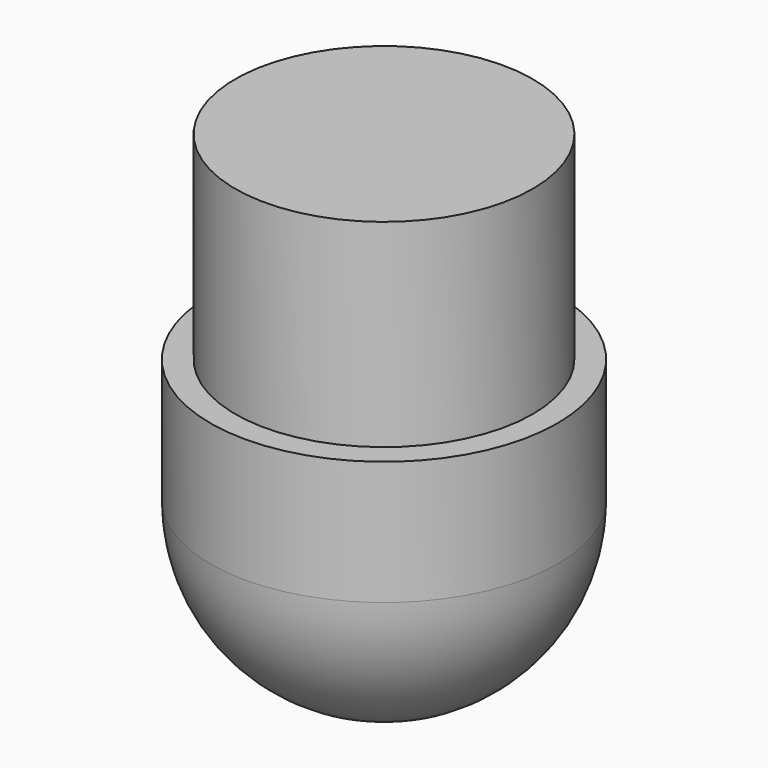
from build123d import *

# Parameters (mm, degrees)
F0_R     = 15
F1_DEPTH = 20
F2_R     = 17.5
F2_R_2   = 15
F3_DEPTH = 30
F5_R     = 17.5


with BuildPart() as f1:
    # F0 (on Top) → F1 (new body)
    with BuildSketch(Plane.XY):
        Circle(F0_R)
    extrude(amount=F1_DEPTH)

    # F2 (on face) → F3 (join)
    with BuildSketch(Plane(origin=(0, 0, 0), x_dir=(1, 0, 0), z_dir=(0, 0, -1))):
        Circle(F2_R)
        Circle(F2_R_2, mode=Mode.SUBTRACT)
        Circle(F2_R_2)
    extrude(amount=F3_DEPTH)

    # F5
    f5_edges = [f1.edges().sort_by_distance(p)[0] for p in [
        (-17.5, 0, -30),
    ]]
    fillet(f5_edges, radius=F5_R)


solid = f1.part
